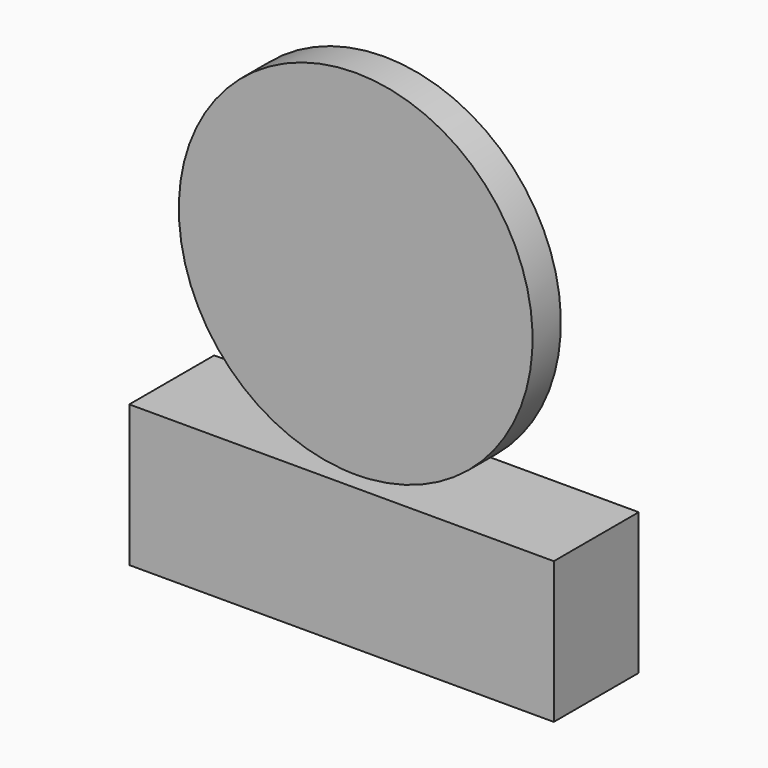
from build123d import *

# Parameters (mm, degrees)
F1_DEPTH = 38.1
F2_DEPTH = 16.51
F3_DEPTH = 25.4


with BuildPart() as f1:
    # F0 (on Front) → F1 (new body, symmetric)
    with BuildSketch(Plane.XZ):
        Polygon((-152.4, -101.6), (152.4, -101.6), (152.4, 0), (9.815774858, 0), (0, 0), (-9.815774858, 0), (-152.4, 0), align=None)
    extrude(amount=F1_DEPTH, both=True)


with BuildPart() as f2:
    # F0 (on Front) → F2 (new body)
    with BuildSketch(Plane.XZ):
        with BuildLine():
            Line((0, 127), (0, 0))
            ThreePointArc((0, 0), (4.9115618074, 0.0950097096), (9.815774858, 0.3798966833))
            Line((9.815774858, 0.3798966833), (9.815774858, 127))
            Line((9.815774858, 127), (0, 127))
        make_face()
        with BuildLine():
            ThreePointArc((-9.815774858, 0.3798966833), (-4.9115618074, 0.0950097096), (0, 0))
            Line((0, 0), (0, 127))
            Line((0, 127), (-9.815774858, 127))
            Line((-9.815774858, 127), (-9.815774858, 0.3798966833))
        make_face()
    extrude(amount=-F2_DEPTH)


with BuildPart() as f3:
    # F0 (on Front) → F3 (new body)
    with BuildSketch(Plane.XZ):
        with BuildLine():
            Line((9.815774858, 127), (9.815774858, 0.3798966833))
            ThreePointArc((9.815774858, 0.3798966833), (93.208377861, 40.7376194595), (127, 127))
            ThreePointArc((127, 127), (-86.2623805405, 220.208377861), (-9.815774858, 0.3798966833))
            Line((-9.815774858, 0.3798966833), (-9.815774858, 127))
            Line((-9.815774858, 127), (0, 127))
            Line((0, 127), (9.815774858, 127))
        make_face()
        with BuildLine():
            ThreePointArc((-9.815774858, 0.3798966833), (-4.9115618074, 0.0950097096), (0, 0))
            Line((0, 0), (0, 127))
            Line((0, 127), (-9.815774858, 127))
            Line((-9.815774858, 127), (-9.815774858, 0.3798966833))
        make_face()
        with BuildLine():
            Line((0, 127), (0, 0))
            ThreePointArc((0, 0), (4.9115618074, 0.0950097096), (9.815774858, 0.3798966833))
            Line((9.815774858, 0.3798966833), (9.815774858, 127))
            Line((9.815774858, 127), (0, 127))
        make_face()
    extrude(amount=F3_DEPTH)


solid = Compound([f1.part, f2.part, f3.part])
